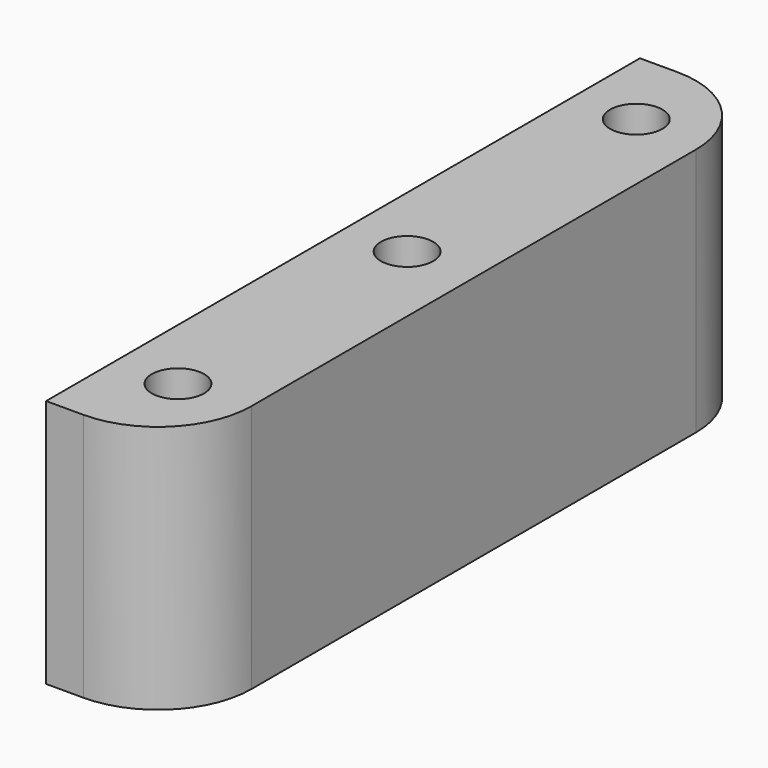
from build123d import *

# Parameters (mm, degrees)
F1_R     = 2.1
F2_DEPTH = 20


# Not quite as in the source:
# - ends of sketch curves that miss each other by under 0.0002 mm in the source are joined


with BuildPart() as f2:
    # F1 (on Top) → F2 (new body)
    with BuildSketch(Plane.XY):
        with BuildLine():
            Line((112.4458007812, 59.6080856323), (109.4554236891, 59.6080856323))
            Line((109.4554236891, 59.6080856323), (109.4554236891, 0))
            Line((109.4554236891, 0), (112.4458007812, 0))
            ThreePointArc((112.4458007812, 0), (117.7491016401, 2.1966991411), (119.9458007812, 7.5))
            add(Edge.make_bspline(
                [(119.9458007812, 52.1080865864), (119.9458007812, 37.238724391), (119.9458007812, 22.3693621955), (119.9458007812, 7.5)],
                knots=[0, 0, 0, 0, 1, 1, 1, 1], degree=3))
            ThreePointArc((119.9458007812, 52.1080865864), (117.7491016401, 57.4113864912), (112.4458007812, 59.6080856323))
        make_face()
        with Locations((114.4458007813, 6.9999980927)):
            Circle(F1_R, mode=Mode.SUBTRACT)
        with Locations((114.4458007813, 29.9999995232)):
            Circle(F1_R, mode=Mode.SUBTRACT)
        with Locations((114.4458007813, 52.9999995232)):
            Circle(F1_R, mode=Mode.SUBTRACT)
    extrude(amount=F2_DEPTH)


solid = f2.part
